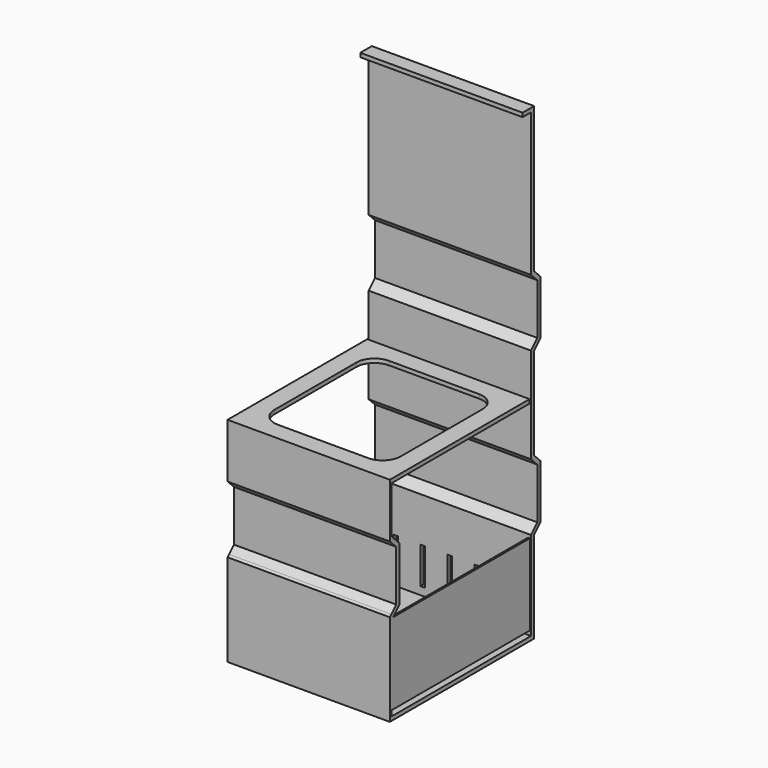
from build123d import *

# Parameters (mm, degrees)
F0_W     = 96.8
F0_H     = 2.2
F0_W_2   = 2.2
F0_W_3   = 1
F0_W_4   = 5.8
F0_W_5   = 95.8395342231
F1_DEPTH = 90
F2_W     = 1
F2_H     = 45
F3_DEPTH = 96
F4_W     = 70
F4_H     = 76.8395342231
F5_DEPTH = 25
F6_R     = 10
F7_W     = 2.5
F7_H     = 20.3
F8_DEPTH = 25


# Not quite as in the source:
# - ends of sketch curves that miss each other by under 0.0002 mm in the source are joined


with BuildPart() as f1:
    # F0 (on Right) → F1 (new body)
    with BuildSketch(Plane.YZ):
        Polygon((-70.5190410137, 78.9974663137), (-66.1190410137, 74.5974663137), (-66.1190410137, 46.4200059881), (-70.5190410137, 42.0200059881), (-70.5190410137, -7.2912638491), (-68.3190410137, -7.2912638491), (-68.3190410137, 41.1087361509), (-63.9190410137, 45.5087361509), (-63.9190410137, 75.5087361509), (-68.3190410137, 79.9087361509), (-68.3190410137, 131.1087361509), (-63.9190410137, 135.5087361509), (-63.9190384975, 165.5087359606), (-68.3190385763, 169.9087361509), (-68.3190385763, 240.5087361509), (-68.3190385763, 248.3087361509), (-70.5190385763, 248.3087361509), (-70.5190385763, 238.3087361509), (-70.5190385763, 168.9974663137), (-66.1190385763, 164.5974663137), (-66.1190410137, 136.4200059881), (-70.5190410137, 132.0200059881), align=None)
        with Locations((-118.9190410137, -8.3912638491)):
            Rectangle(F0_W, F0_H)
        with Locations((-69.4190410137, -8.3912638491)):
            Rectangle(F0_W_2, F0_H)
        Polygon((-168.3190410137, -7.2912638491), (-167.3190410137, -7.2912638491), (-167.3190410137, 39.4887340454), (-168.3190410137, 38.4768152958), align=None)
        with Locations((-167.8190410137, -8.3912638491)):
            Rectangle(F0_W_3, F0_H)
        Polygon((-168.3190410137, 38.4768152958), (-167.3190410137, 39.4887340454), (-167.3190410137, 42.6143072478), (-168.3190410137, 41.6143048104), align=None)
        Polygon((-167.3190410137, 42.6143072478), (-167.3190410137, 39.4887340454), (-166.1190411219, 40.7030364356), (-161.7190464841, 45.1030417978), (-161.7190408009, 75.1030386029), (-166.1190410137, 79.5030349731), (-167.3190410137, 80.7030349731), (-167.3190410137, 77.5917651359), (-163.9190410137, 74.1917651359), (-163.9190475947, 46.0143089539), align=None)
        with Locations((-73.4190385763, 249.4087361509)):
            Rectangle(F0_W_4, F0_H)
        with Locations((-69.4190385763, 249.4087361509)):
            Rectangle(F0_W_2, F0_H)
        Polygon((-168.3190410137, 78.5917651359), (-167.3190410137, 77.5917651359), (-167.3190410137, 80.7030349731), (-168.3190410137, 81.7030349731), align=None)
        Polygon((-168.3190410137, 81.7030349731), (-167.3190410137, 80.7030349731), (-167.3190410137, 106.5323576331), (-168.3190410137, 106.5323576331), align=None)
        with Locations((-167.8190410137, 107.6323576331)):
            Rectangle(F0_W_3, F0_H)
        with Locations((-119.3992739022, 107.6323576331)):
            Rectangle(F0_W_5, F0_H)
    extrude(amount=F1_DEPTH)

    # F2 (on face) → F3 (join)
    with BuildSketch(Plane(origin=(0, -167.3190410137, 0), x_dir=(-1, 0, 0), z_dir=(0, 1, 0))):
        with Locations((-89.5, 18.2087361509)):
            Rectangle(F2_W, F2_H)
        with Locations((-0.5, 18.2087361509)):
            Rectangle(F2_W, F2_H)
    extrude(amount=F3_DEPTH)

    # F4 (on face) → F5 (cut)
    with BuildSketch(Plane.XY.offset(108.7323576331)):
        with Locations((45, -119.8992739022)):
            Rectangle(F4_W, F4_H)
    extrude(amount=-F5_DEPTH, mode=Mode.SUBTRACT)

    # F6
    f6_edges = [f1.edges().sort_by_distance(p)[0] for p in [
        (10, -81.479507, 107.632358),
        (10, -158.319041, 107.632358),
        (80, -81.479507, 107.632358),
        (80, -158.319041, 107.632358),
    ]]
    fillet(f6_edges, radius=F6_R)

    # F7 (on face) → F8 (cut)
    with BuildSketch(Plane(origin=(0, -68.3190410137, 0), x_dir=(-1, 0, 0), z_dir=(0, 1, 0))):
        with Locations((-75, 7.2530107699)):
            Rectangle(F7_W, F7_H)
        with Locations((-60, 7.2530107699)):
            Rectangle(F7_W, F7_H)
        with Locations((-45, 7.2530107699)):
            Rectangle(F7_W, F7_H)
        with Locations((-30, 7.2530107699)):
            Rectangle(F7_W, F7_H)
        with Locations((-15, 7.2530107699)):
            Rectangle(F7_W, F7_H)
    extrude(amount=-F8_DEPTH, mode=Mode.SUBTRACT)


solid = f1.part
